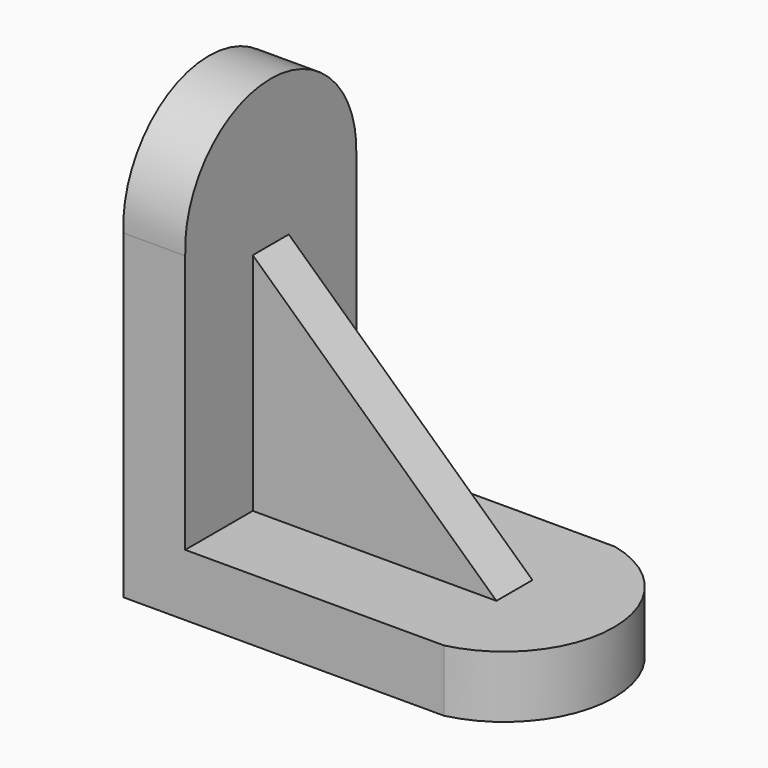
from build123d import *

# Parameters (mm, degrees)
F1_DEPTH = 38
F2_W     = 8
F2_H     = 40
F3_DEPTH = 43.3
F5_DEPTH = 11
F7_DEPTH = 11
F9_DEPTH = 42.4


with BuildPart() as f1:
    # F0 (on Front) → F1 (new body)
    with BuildSketch(Plane.XZ):
        Polygon((-20.403226763, 14.420258379), (-31.403226763, 14.420258379), (-31.403226763, -42.579741621), (25.596773237, -42.579741621), (25.596773237, -31.579741621), (-20.403226763, -31.579741621), align=None)
    extrude(amount=-F1_DEPTH)

    # F2 (on face) → F3 (join)
    with BuildSketch(Plane.YZ.offset(-20.403226763)):
        Polygon((23, -31.579741621), (15, -31.579741621), (26, -37.2273437679), (34.1856418401, -37.2273437679), align=None)
        with Locations((19, -11.579741621)):
            Rectangle(F2_W, F2_H)
    extrude(amount=F3_DEPTH)

    # F4 (on face) → F5 (join)
    with BuildSketch(Plane.XY.offset(-31.579741621)):
        with BuildLine():
            Line((25.596773237, 38), (25.596773237, 0))
            ThreePointArc((25.596773237, 0), (40.596773237, 19), (25.596773237, 38))
        make_face()
    extrude(amount=-F5_DEPTH)

    # F6 (on face) → F7 (join)
    with BuildSketch(Plane.YZ.offset(-20.403226763)):
        with BuildLine():
            Line((0, 14.420258379), (38, 14.420258379))
            ThreePointArc((38, 14.420258379), (19, 34.420258379), (0, 14.420258379))
        make_face()
    extrude(amount=-F7_DEPTH)

    # F8 (on face) → F9 (cut)
    with BuildSketch(Plane.XZ.offset(-15)):
        Polygon((22.896773237, 8.420258379), (-20.403226763, 8.420258379), (22.896773237, -31.579741621), align=None)
    extrude(amount=-F9_DEPTH, mode=Mode.SUBTRACT)


solid = f1.part
